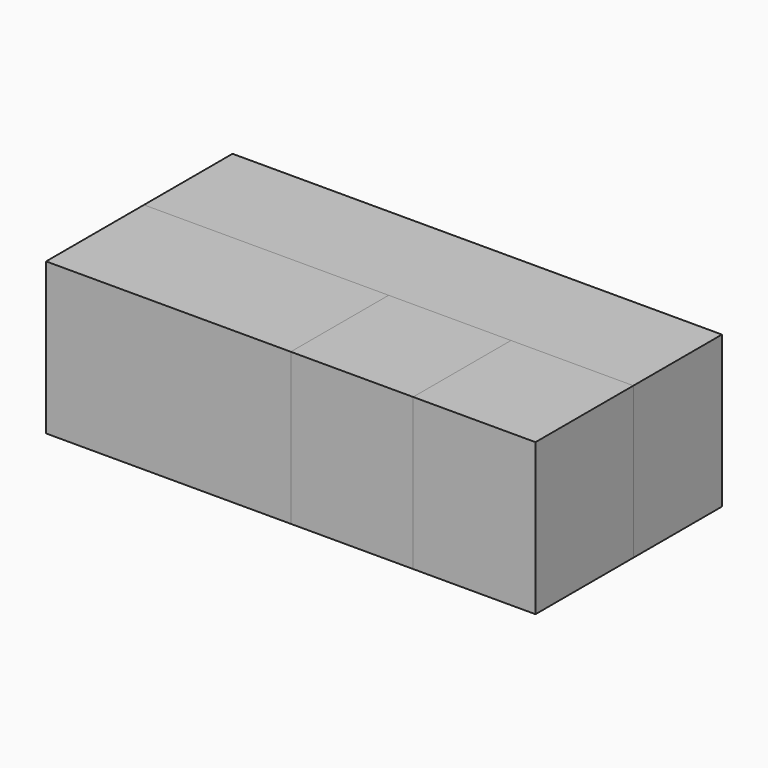
from build123d import *

# Parameters (mm, degrees)
F0_W      = 47.5
F0_H      = 65
F0_W_2    = 52.5
F1_DEPTH  = 210
F2_DEPTH  = 105
F3_DEPTH  = 157.5
F4_DEPTH  = 52.5
F5_DEPTH  = 210
F6_W      = 105
F6_H      = 52.5
F7_DEPTH  = 65.001
F8_DEPTH  = 105
F9_W      = 105
F9_H      = 52.5
F10_DEPTH = 65.001
F11_DEPTH = 210
F12_DEPTH = 157.5
F13_DEPTH = 210


with BuildPart() as f1:
    # F0 (on Right) → F1 (new body)
    with BuildSketch(Plane.YZ):
        with Locations((26.25, 0)):
            Rectangle(F0_W, F0_H)
        with Locations((-23.75, 0)):
            Rectangle(F0_W_2, F0_H)
    extrude(amount=F1_DEPTH)


with BuildPart() as f2:
    # F0 (on Right) → F2 (new body)
    with BuildSketch(Plane.YZ):
        with Locations((26.25, 0)):
            Rectangle(F0_W, F0_H)
        with Locations((-23.75, 0)):
            Rectangle(F0_W_2, F0_H)
    extrude(amount=F2_DEPTH)


with BuildPart() as f3:
    # F0 (on Right) → F3 (new body)
    with BuildSketch(Plane.YZ):
        with Locations((26.25, 0)):
            Rectangle(F0_W, F0_H)
        with Locations((-23.75, 0)):
            Rectangle(F0_W_2, F0_H)
    extrude(amount=F3_DEPTH)


with BuildPart() as f4:
    # F0 (on Right) → F4 (new body)
    with BuildSketch(Plane.YZ):
        with Locations((26.25, 0)):
            Rectangle(F0_W, F0_H)
        with Locations((-23.75, 0)):
            Rectangle(F0_W_2, F0_H)
    extrude(amount=F4_DEPTH)


with BuildPart() as f5:
    # F0 (on Right) → F5 (new body)
    with BuildSketch(Plane.YZ):
        with Locations((26.25, 0)):
            Rectangle(F0_W, F0_H)
        with Locations((-23.75, 0)):
            Rectangle(F0_W_2, F0_H)
    extrude(amount=F5_DEPTH)

    # F6 (on face) → F7 (cut, through all)
    with BuildSketch(Plane.XY.offset(32.5)):
        with Locations((157.5, -23.75)):
            Rectangle(F6_W, F6_H)
    extrude(amount=-F7_DEPTH, mode=Mode.SUBTRACT)


with BuildPart() as f8:
    # F0 (on Right) → F8 (new body)
    with BuildSketch(Plane.YZ):
        with Locations((26.25, 0)):
            Rectangle(F0_W, F0_H)
        with Locations((-23.75, 0)):
            Rectangle(F0_W_2, F0_H)
    extrude(amount=F8_DEPTH)

    # F9 (on face) → F10 (cut, through all)
    with BuildSketch(Plane.XY.offset(32.5)):
        with Locations((52.5, -23.75)):
            Rectangle(F9_W, F9_H)
    extrude(amount=-F10_DEPTH, mode=Mode.SUBTRACT)


with BuildPart() as f11:
    # F0 (on Right) → F11 (new body)
    with BuildSketch(Plane.YZ):
        with Locations((26.25, 0)):
            Rectangle(F0_W, F0_H)
    extrude(amount=F11_DEPTH)


with BuildPart() as f12:
    # F0 (on Right) → F12 (new body)
    with BuildSketch(Plane.YZ):
        with Locations((26.25, 0)):
            Rectangle(F0_W, F0_H)
    extrude(amount=F12_DEPTH)


with BuildPart() as f13:
    # F0 (on Right) → F13 (new body)
    with BuildSketch(Plane.YZ):
        with Locations((26.25, 0)):
            Rectangle(F0_W, F0_H)
    extrude(amount=F13_DEPTH)


solid = Compound([f1.part, f2.part, f3.part, f4.part, f5.part, f8.part, f11.part, f12.part, f13.part])
